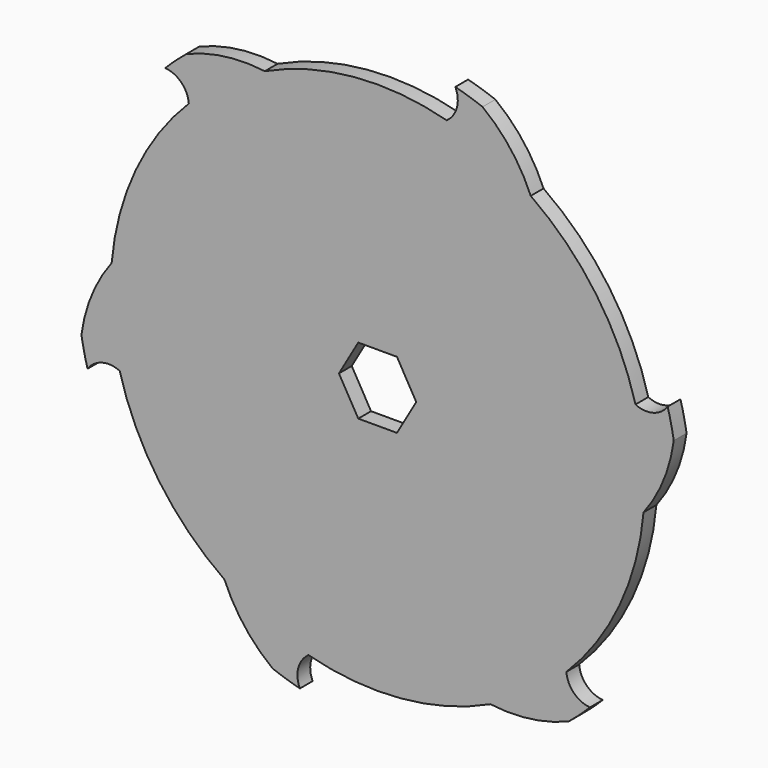
from build123d import *

# Parameters (mm, degrees)
F0_R            = 50.00625
F1_DEPTH        = 1.3335
F3_DEPTH        = 25.4
F3_DEPTH_BACK   = 25.4
F3_COPIES_COUNT = 6


# Not quite as in the source:
# - a pattern or mirror of a feature is missing from the dataset's text; its kind, count and spacing are read off the source's solid


with BuildPart() as f1:
    # F0 (on Front) → F1 (new body, symmetric)
    with BuildSketch(Plane.XZ):
        Circle(F0_R)
        Polygon((-6.4378019116, 0), (-3.2189009558, 5.5753), (3.2189009558, 5.5753), (6.4378019116, 0), (3.2189009558, -5.5753), (-3.2189009558, -5.5753), align=None, mode=Mode.SUBTRACT)
    extrude(amount=F1_DEPTH, both=True)

    # F2 (on Front) → F3 (cut, two sides)
    with BuildSketch(Plane.XZ) as f3_sk:
        with BuildLine():
            ThreePointArc((-18.7853817344, 40.2853811338), (-3.8740727651, 44.2808543302), (11.5045065548, 42.9354029785))
            ThreePointArc((11.5045065548, 42.9354029785), (13.205652236, 45.3557090058), (12.9425698742, 48.3023283509))
            ThreePointArc((12.9425698742, 48.3023283509), (-10.6277765567, 48.8638455765), (-31.8356210179, 38.5631725026))
            ThreePointArc((-31.8356210179, 38.5631725026), (-25.4240052006, 40.2843654517), (-18.7853817344, 40.2853811338))
        make_face()
    f3 = extrude(amount=-F3_DEPTH, mode=Mode.SUBTRACT) + extrude(f3_sk.sketch, amount=F3_DEPTH_BACK, mode=Mode.SUBTRACT)

    # F3_copies: F3 ×6 about axis
    f3_copies_axis = Axis((0, 0, 0), (0, 1, 0))
    for i in range(1, F3_COPIES_COUNT):
        add(f3.rotate(f3_copies_axis, i * 360 / F3_COPIES_COUNT), mode=Mode.SUBTRACT)


solid = f1.part
